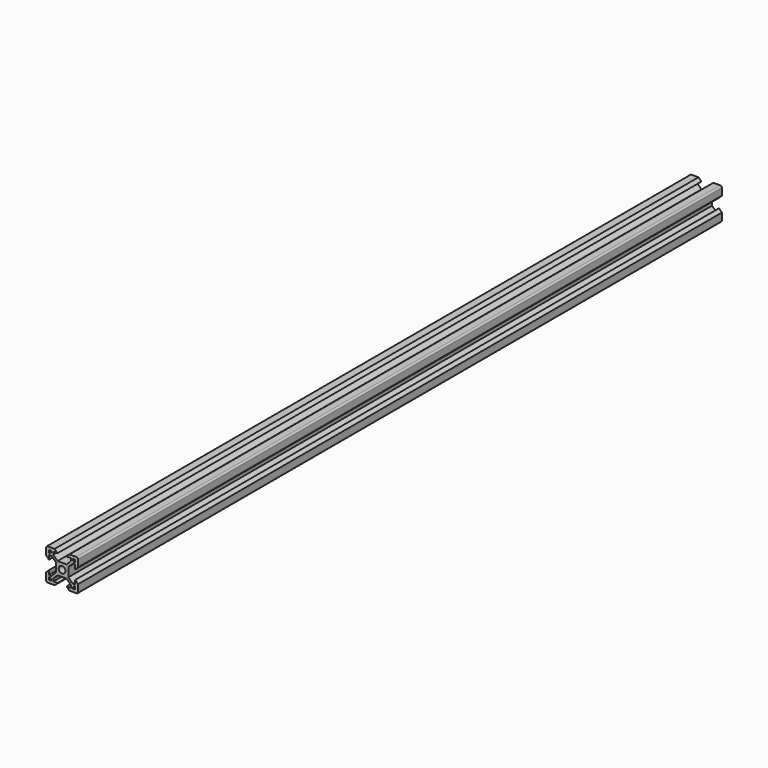
from build123d import *

# Parameters (mm, degrees)
F0_W            = 20
F0_H            = 20
F1_DEPTH        = 503
F2_R            = 2.1
F3_DEPTH        = 503.001
F4_R            = 1
F6_DEPTH        = 503.001
F6_COPIES_COUNT = 4


# Not quite as in the source:
# - a pattern or mirror of a feature is missing from the dataset's text; its kind, count and spacing are read off the source's solid


with BuildPart() as f1:
    # F0 (on Front) → F1 (new body)
    with BuildSketch(Plane.XZ):
        Rectangle(F0_W, F0_H)
    extrude(amount=F1_DEPTH)

    # F2 (on face) → F3 (cut, through all)
    with BuildSketch(Plane.XZ.offset(503)):
        Circle(F2_R)
    extrude(amount=-F3_DEPTH, mode=Mode.SUBTRACT)

    # F4
    f4_edges = [f1.edges().sort_by_distance(p)[0] for p in [
        (-10, -251.5, 10),
        (10, -251.5, 10),
        (10, -251.5, -10),
        (-10, -251.5, -10),
    ]]
    fillet(f4_edges, radius=F4_R)

    # F5 (on face) → F6 (cut, through all)
    with BuildSketch(Plane.XZ.offset(503)):
        Polygon((0, 3.9006601718), (0, 10), (-2.84, 10), (-4.64, 10), (-2.84, 8.2), (-5.4993398282, 8.2), (-5.4993398282, 6.56), (-2.84, 3.9006601718), align=None)
        Polygon((-6.5693398282, 8.2), (-8.2, 8.2), (-7.0953059148, 7.0953059148), (-6.5693398282, 7.6212720014), align=None)
    f6 = extrude(amount=-F6_DEPTH, mode=Mode.SUBTRACT)

    # F6_copies: F6 ×4 about axis
    f6_copies_axis = Axis((0, 0, 0), (0, 1, 0))
    for i in range(1, F6_COPIES_COUNT):
        add(f6.rotate(f6_copies_axis, i * 360 / F6_COPIES_COUNT), mode=Mode.SUBTRACT)

    # F6_copies1: F6 across plane
    add(f6.mirror(Plane(origin=(0, 0, 0), x_dir=(-0.7071067812, 0, -0.7071067812), z_dir=(0.7071067812, 0, -0.7071067812))), mode=Mode.SUBTRACT)

    # F6_copies2: F6 across plane
    add(f6.mirror(Plane(origin=(0, 0, 0), x_dir=(-1, 0, 0), z_dir=(0, 0, -1))), mode=Mode.SUBTRACT)

    # F6_copies3: F6 across plane
    add(f6.mirror(Plane(origin=(0, 0, 0), x_dir=(0, 0, 1), z_dir=(1, 0, 0))), mode=Mode.SUBTRACT)

    # F6_copies4: F6 across plane
    add(f6.mirror(Plane(origin=(0, 0, 0), x_dir=(0.7071067812, 0, -0.7071067812), z_dir=(-0.7071067812, 0, -0.7071067812))), mode=Mode.SUBTRACT)


solid = f1.part
